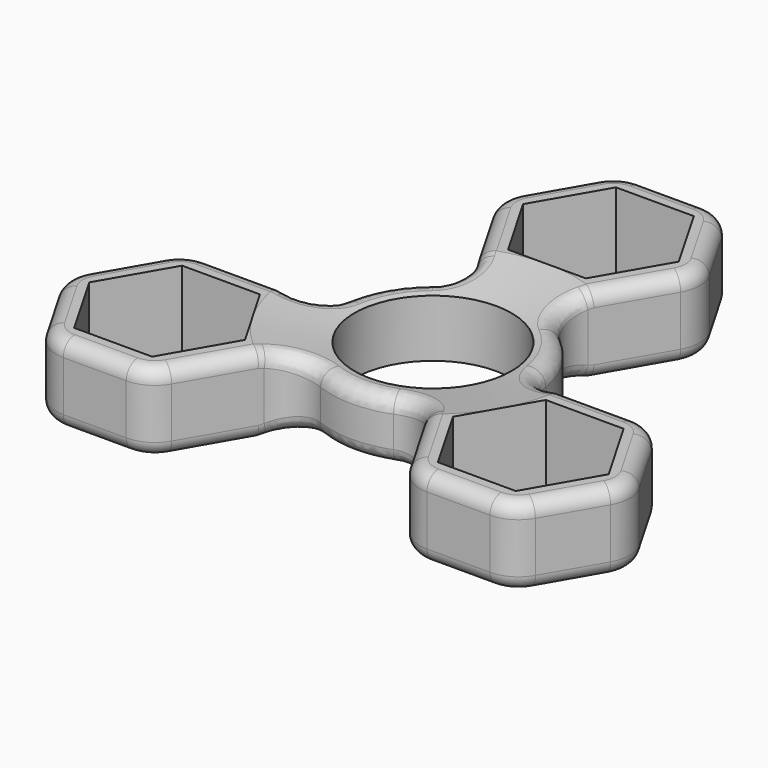
from build123d import *

# Parameters (mm, degrees)
F0_R     = 10.95
F1_DEPTH = 5.5
F4_R     = 5
F5_R     = 2


with BuildPart() as f1:
    # F0 (on Top) → F1 (new body, symmetric)
    with BuildSketch(Plane.XY):
        with BuildLine():
            Line((7.2746133918, 16.6727835234), (14.5492267836, 29.2727835234))
            Line((14.5492267836, 29.2727835234), (7.2746133918, 41.8727835234))
            Line((7.2746133918, 41.8727835234), (-7.2746133918, 41.8727835234))
            Line((-7.2746133918, 41.8727835234), (-14.5492267836, 29.2727835234))
            Line((-14.5492267836, 29.2727835234), (-7.2746133918, 16.6727835234))
            Line((-7.2746133918, 16.6727835234), (-5.2377830256, 13.1448898427))
            ThreePointArc((-5.2377830256, 13.1448898427), (-12.2542594635, 7.075), (-14.0027000465, -2.0363917617))
            Line((-14.0027000465, -2.0363917617), (-18.076360779, -2.0363917617))
            Line((-18.076360779, -2.0363917617), (-32.6255875626, -2.0363917617))
            Line((-32.6255875626, -2.0363917617), (-39.9002009544, -14.6363917617))
            Line((-39.9002009544, -14.6363917617), (-32.6255875626, -27.2363917617))
            Line((-32.6255875626, -27.2363917617), (-18.076360779, -27.2363917617))
            Line((-18.076360779, -27.2363917617), (-10.8017473872, -14.6363917617))
            Line((-10.8017473872, -14.6363917617), (-8.764917021, -11.108498081))
            ThreePointArc((-8.764917021, -11.108498081), (0, -14.15), (8.764917021, -11.108498081))
            Line((8.764917021, -11.108498081), (10.8017473872, -14.6363917617))
            Line((10.8017473872, -14.6363917617), (18.076360779, -27.2363917617))
            Line((18.076360779, -27.2363917617), (32.6255875626, -27.2363917617))
            Line((32.6255875626, -27.2363917617), (39.9002009544, -14.6363917617))
            Line((39.9002009544, -14.6363917617), (32.6255875626, -2.0363917617))
            Line((32.6255875626, -2.0363917617), (18.076360779, -2.0363917617))
            Line((18.076360779, -2.0363917617), (14.0027000465, -2.0363917617))
            ThreePointArc((14.0027000465, -2.0363917617), (12.2542594636, 7.075), (5.2377830256, 13.1448898427))
            Line((5.2377830256, 13.1448898427), (7.2746133918, 16.6727835234))
        make_face()
        Polygon((-19.9238816404, -5.2363917617), (-14.49678911, -14.6363917617), (-19.9238816404, -24.0363917617), (-30.7780667012, -24.0363917617), (-36.2051592315, -14.6363917617), (-30.7780667012, -5.2363917617), align=None, mode=Mode.SUBTRACT)
        Polygon((30.7780667012, -5.2363917617), (36.2051592315, -14.6363917617), (30.7780667012, -24.0363917617), (19.9238816404, -24.0363917617), (14.49678911, -14.6363917617), (19.9238816404, -5.2363917617), align=None, mode=Mode.SUBTRACT)
        Circle(F0_R, mode=Mode.SUBTRACT)
        Polygon((5.4270925304, 38.6727835234), (10.8541850608, 29.2727835234), (5.4270925304, 19.8727835234), (-5.4270925304, 19.8727835234), (-10.8541850608, 29.2727835234), (-5.4270925304, 38.6727835234), align=None, mode=Mode.SUBTRACT)
    extrude(amount=F1_DEPTH, both=True)

    # F2 (on Right) → F3 (revolve, cut)
    with BuildSketch(Plane.YZ):
        Polygon((10.95, 5.5), (10.95, 4), (19.8727835234, 5.5), align=None)
        Polygon((19.8727835234, -5.5), (10.95, -4), (10.95, -5.5), align=None)
    revolve(axis=Axis((0, 0, 6.7626568489), (0, 0, 1)), mode=Mode.SUBTRACT)

    # F4
    f4_edges = [f1.edges().sort_by_distance(p)[0] for p in [
        (-5.237783, 13.14489, 0),
        (-14.0027, -2.036392, 0),
        (8.764917, -11.108498, 0),
        (-8.764917, -11.108498, 0),
        (14.0027, -2.036392, 0),
        (5.237783, 13.14489, 0),
        (32.625588, -2.036392, 0),
        (39.900201, -14.636392, 0),
        (32.625588, -27.236392, 0),
        (18.076361, -27.236392, 0),
        (-18.076361, -27.236392, 0),
        (-32.625588, -27.236392, 0),
        (-39.900201, -14.636392, 0),
        (-32.625588, -2.036392, 0),
        (-14.549227, 29.272784, 0),
        (-7.274613, 41.872784, 0),
        (7.274613, 41.872784, 0),
        (14.549227, 29.272784, 0),
    ]]
    fillet(f4_edges, radius=F4_R)

    # F5
    f5_edges = [f1.edges().sort_by_distance(p)[0] for p in [
        (-25.350974, -27.236392, 5.5),
        (-25.350974, -27.236392, -5.5),
        (-12.254259, 7.075, 4.537949),
        (-10.91192, 35.572784, 5.5),
        (12.254259, 7.075, 4.537949),
        (36.262894, -20.936392, 5.5),
        (0, -14.15, 4.537949),
        (0, -14.15, -4.537949),
        (36.262894, -20.936392, -5.5),
        (0, 41.872784, -5.5),
        (12.254259, 7.075, -4.537949),
        (-12.254259, 7.075, -4.537949),
    ]]
    fillet(f5_edges, radius=F5_R)


solid = f1.part
